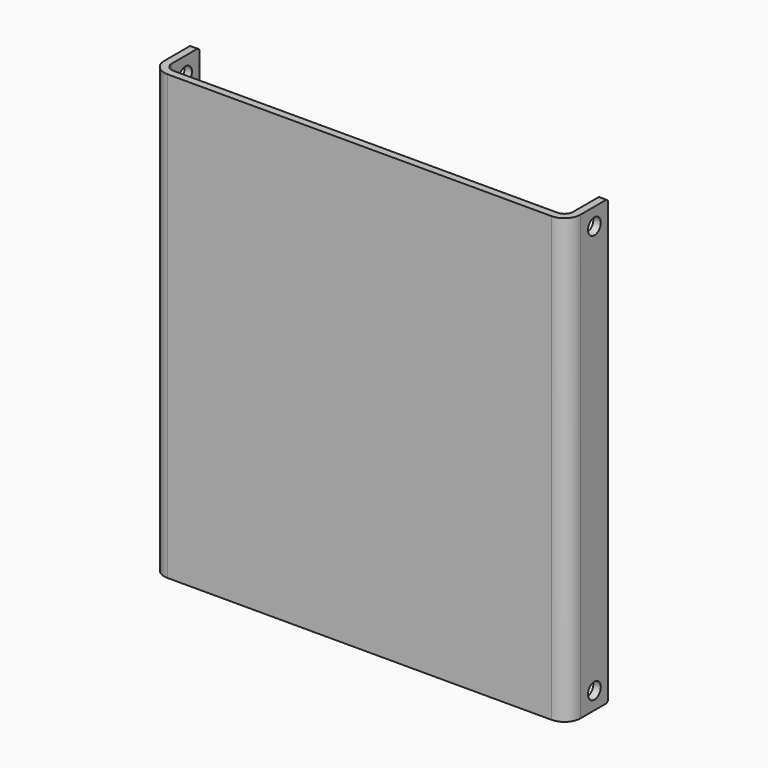
from build123d import *

# Parameters (mm, degrees)
F1_DEPTH = 101.6
F2_R     = 3.69316
F3_R     = 1.98374
F4_R     = 1.8288
F5_DEPTH = 95.37192
F6_R     = 0.762


with BuildPart() as f1:
    # F0 (on Top) → F1 (new body)
    with BuildSketch(Plane.XY):
        Polygon((0, 9.92124), (0, 0), (-91.95308, 0), (-91.95308, 9.92124), (-93.6625, 9.92124), (-93.6625, -1.70942), (1.70942, -1.70942), (1.70942, 9.92124), align=None)
    extrude(amount=F1_DEPTH)

    # F2
    f2_edges = [f1.edges().sort_by_distance(p)[0] for p in [
        (1.70942, -1.70942, 50.8),
        (-93.6625, -1.70942, 50.8),
    ]]
    fillet(f2_edges, radius=F2_R)

    # F3
    f3_edges = [f1.edges().sort_by_distance(p)[0] for p in [
        (0, 0, 50.8),
        (-91.95308, 0, 50.8),
    ]]
    fillet(f3_edges, radius=F3_R)

    # F4 (on face) → F5 (cut, through all)
    with BuildSketch(Plane.YZ.offset(1.70942)):
        with Locations((5.95249, 97.63125)):
            Circle(F4_R)
        with Locations((5.95249, 3.96875)):
            Circle(F4_R)
    extrude(amount=-F5_DEPTH, mode=Mode.SUBTRACT)

    # F6
    f6_edges = [f1.edges().sort_by_distance(p)[0] for p in [
        (-92.80779, 9.92124, 101.6),
        (-92.80779, 9.92124, 0),
        (0.85471, 9.92124, 0),
        (0.85471, 9.92124, 101.6),
    ]]
    fillet(f6_edges, radius=F6_R)


solid = f1.part
